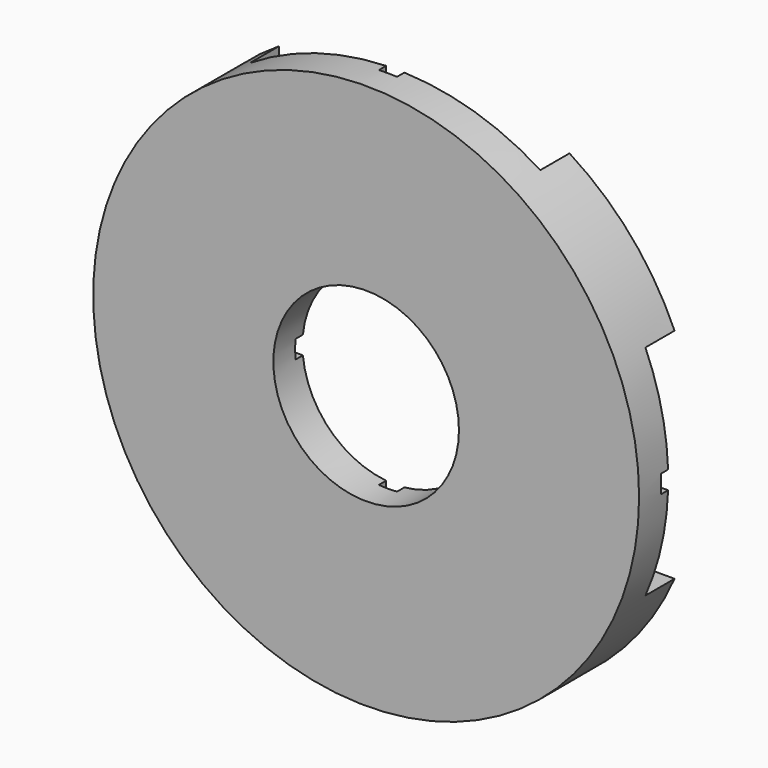
from build123d import *

# Parameters (mm, degrees)
F0_R          = 12.7
F1_DEPTH      = 17.78
F2_R          = 38.1
F3_DEPTH      = 10.16
F4_R          = 12.954
F5_DEPTH      = 17.781
F5_DEPTH_BACK = 115
F6_W          = 5.08
F6_H          = 30.48
F7_DEPTH      = 38.101
F7_DEPTH_BACK = 38.101
F8_W          = 40.513
F8_H          = 5.08
F9_DEPTH      = 38.101
F9_DEPTH_BACK = 38.101
F11_DEPTH     = 6.35


# Not quite as in the source:
# - an extrude ends at something that could not be found from the text; its depth is read off the source's solid


with BuildPart() as f1:
    # F0 (on Front) → F1 (new body)
    with BuildSketch(Plane.XZ):
        Circle(F0_R)
    extrude(amount=F1_DEPTH)

    # F2 (on Front) → F3 (join)
    with BuildSketch(Plane.XZ):
        Circle(F2_R)
    extrude(amount=F3_DEPTH)

    # F4 (on Front) → F5 (cut, two sides)
    with BuildSketch(Plane.XZ) as f5_sk:
        Circle(F4_R)
    extrude(amount=F5_DEPTH, mode=Mode.SUBTRACT)
    extrude(f5_sk.sketch, amount=-F5_DEPTH_BACK, mode=Mode.SUBTRACT)

    # F6 (on Right) → F7 (cut, two sides)
    with BuildSketch(Plane.YZ) as f7_sk:
        with Locations((-2.54, 0)):
            Rectangle(F6_W, F6_H)
    extrude(amount=F7_DEPTH, mode=Mode.SUBTRACT)
    extrude(f7_sk.sketch, amount=-F7_DEPTH_BACK, mode=Mode.SUBTRACT)

    # F8 (on Top) → F9 (cut, two sides)
    with BuildSketch(Plane.XY) as f9_sk:
        with Locations((0, -2.54)):
            Rectangle(F8_W, F8_H)
    extrude(amount=-F9_DEPTH, mode=Mode.SUBTRACT)
    extrude(f9_sk.sketch, amount=F9_DEPTH_BACK, mode=Mode.SUBTRACT)

    # F10 (on face) → F11 (cut)
    with BuildSketch(Plane(origin=(0, 0, 0), x_dir=(-1, 0, 0), z_dir=(0, 1, 0))):
        with BuildLine():
            Line((1.27, -1.27), (38.0788274504, -1.27))
            ThreePointArc((38.0788274504, -1.27), (38.1, 0), (38.0788274504, 1.27))
            Line((38.0788274504, 1.27), (1.27, 1.27))
            Line((1.27, 1.27), (1.27, 38.0788274504))
            ThreePointArc((1.27, 38.0788274504), (0, 38.1), (-1.27, 38.0788274504))
            Line((-1.27, 38.0788274504), (-1.27, 1.27))
            Line((-1.27, 1.27), (-38.0788274504, 1.27))
            ThreePointArc((-38.0788274504, 1.27), (-38.1, 0), (-38.0788274504, -1.27))
            Line((-38.0788274504, -1.27), (-1.27, -1.27))
            Line((-1.27, -1.27), (-1.27, -38.0788274504))
            ThreePointArc((-1.27, -38.0788274504), (0, -38.1), (1.27, -38.0788274504))
            Line((1.27, -38.0788274504), (1.27, -1.27))
        make_face()
    extrude(amount=-F11_DEPTH, mode=Mode.SUBTRACT)


solid = f1.part
